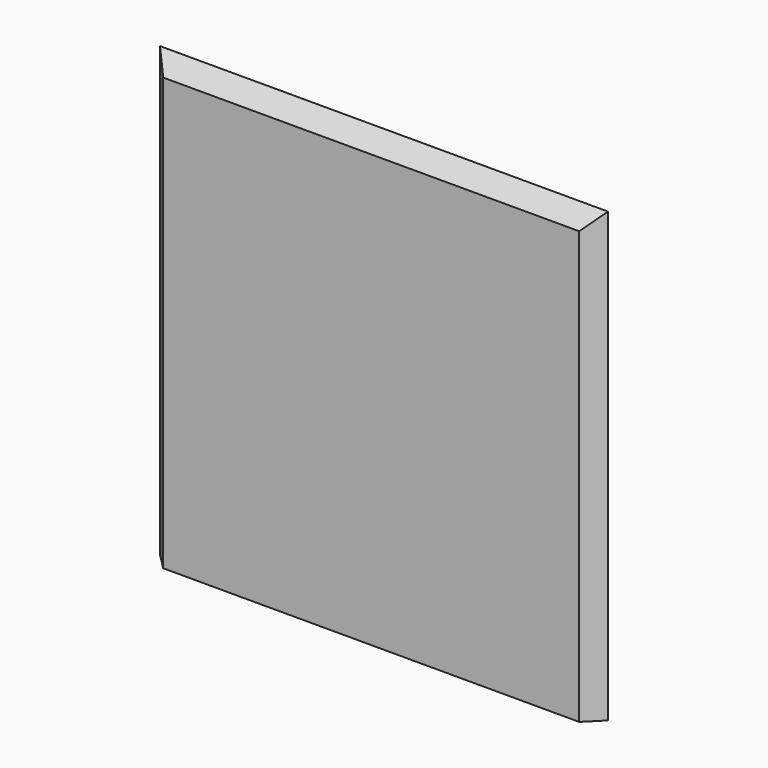
from build123d import *

# Parameters (mm, degrees)
F0_W     = 533.4
F0_H     = 533.4
F1_DEPTH = 19.05
F2_SIZE  = 19.04999


# Not quite as in the source:
# - a fillet or chamfer is up to 0.001 mm smaller than in the source, because OpenCascade refuses the exact size


with BuildPart() as f1:
    # F0 (on Front) → F1 (new body)
    with BuildSketch(Plane.XZ):
        with Locations((1.6536265612, 65.1198284748)):
            Rectangle(F0_W, F0_H)
    extrude(amount=F1_DEPTH)

    # F2 (size 19.05 in the source; OpenCascade refuses exactly that, so slightly less here)
    f2_edges = [f1.edges().sort_by_distance(p)[0] for p in [
        (1.653627, -19.05, 331.819828),
        (-265.046373, -19.05, 65.119828),
        (268.353627, -19.05, 65.119828),
    ]]
    chamfer(f2_edges, length=F2_SIZE)


solid = f1.part
